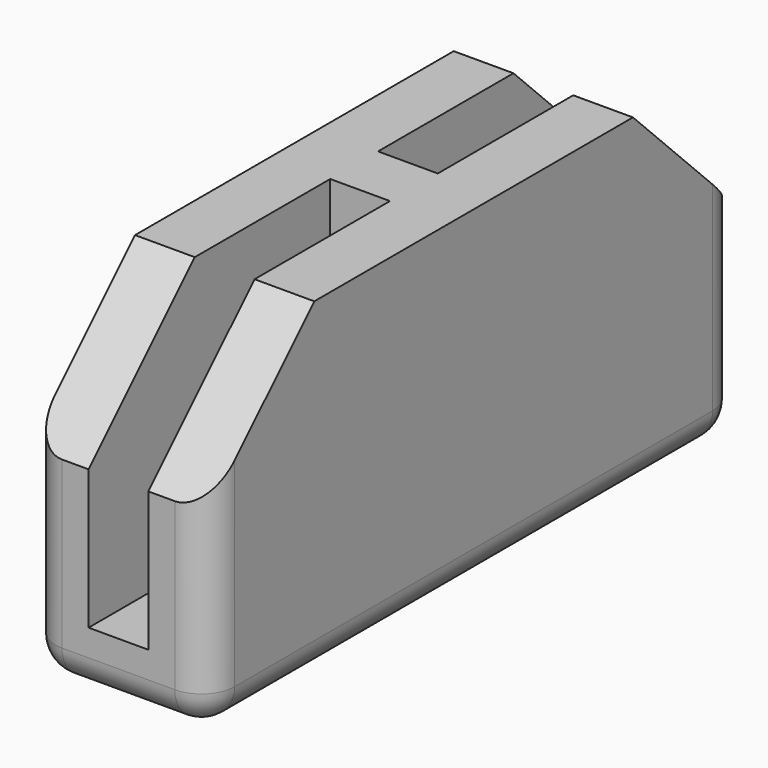
from build123d import *

# Parameters (mm, degrees)
F0_W      = 41
F0_H      = 9
F1_DEPTH  = 41
F3_DEPTH  = 9
F5_DEPTH  = 9
F7_DEPTH  = 30
F9_DEPTH  = 30
F11_DEPTH = 9
F13_DEPTH = 25
F14_R     = 1
F16_W     = 18
F16_H     = 9
F17_DEPTH = 41
F19_DEPTH = 50.001
F20_R     = 5
F21_W     = 9
F21_H     = 41
F22_DEPTH = 30
F23_W     = 27
F23_H     = 9
F24_DEPTH = 41


with BuildPart() as f1:
    # F0 (on Top) → F1 (new body)
    with BuildSketch(Plane.XY):
        Polygon((0, 50), (0, 0), (27, 0), (27, 4.5), (27, 13.5), (27, 22.5), (27, 50), (18, 50), (18, 4.5), (9, 4.5), (9, 50), align=None)
        with Locations((47.5, 9)):
            Rectangle(F0_W, F0_H)
    extrude(amount=F1_DEPTH)

    # F2 (on Top) → F3 (join)
    with BuildSketch(Plane.XY):
        Polygon((0, 50), (0, 0), (68, 0), (68, 13.5), (27, 50), align=None)
    extrude(amount=-F3_DEPTH)

    # F4 (on face) → F5 (cut, through all)
    with BuildSketch(Plane.XY):
        Polygon((56.1775657399, 18), (31.5, 39.9690524269), (31.5, 18), align=None)
    extrude(amount=-F5_DEPTH, mode=Mode.SUBTRACT)

    # F6 (on face) → F7 (cut)
    with BuildSketch(Plane(origin=(0, 0, 0), x_dir=(0, -1, 0), z_dir=(-1, 0, 0))):
        Polygon((-50, 21), (-30, 41), (-50, 41), align=None)
    extrude(amount=-F7_DEPTH, mode=Mode.SUBTRACT)

    # F8 (on face) → F9 (cut)
    with BuildSketch(Plane.XZ):
        Polygon((0, 21), (0, 41), (-20, 41), align=None)
    extrude(amount=-F9_DEPTH, mode=Mode.SUBTRACT)

    # F10 (on face) → F11 (cut, through all)
    with BuildSketch(Plane.XY):
        with BuildLine():
            Line((9, 36.5), (9, 13.5))
            ThreePointArc((9, 13.5), (10.3180194847, 10.3180194847), (13.5, 9))
            ThreePointArc((13.5, 9), (16.6819805153, 10.3180194847), (18, 13.5))
            Line((18, 13.5), (18, 36.5))
            ThreePointArc((18, 36.5), (16.6819805153, 39.6819805153), (13.5, 41))
            ThreePointArc((13.5, 41), (10.3180194847, 39.6819805153), (9, 36.5))
        make_face()
        with BuildLine():
            ThreePointArc((59, 0), (57.6819805153, 3.1819805153), (54.5, 4.5))
            Line((54.5, 4.5), (40.5, 4.5))
            ThreePointArc((40.5, 4.5), (37.3180194847, 3.1819805153), (36, 0))
            Line((36, 0), (59, 0))
        make_face()
    extrude(amount=-F11_DEPTH, mode=Mode.SUBTRACT)

    # F12 (on face) → F13 (cut)
    with BuildSketch(Plane.XZ.offset(-4.5)):
        Polygon((68, 21), (68, 41), (48, 41), align=None)
        Polygon((59, 17.2720779386), (44.2720779386, 32), (36, 32), (36, 9), (59, 9), align=None)
    extrude(amount=-F13_DEPTH, mode=Mode.SUBTRACT)

    # F14
    f14_edges = [f1.edges().sort_by_distance(p)[0] for p in [
        (31.5, 18, -4.5),
        (31.5, 39.969052, -4.5),
        (56.177566, 18, -4.5),
        (36, 9, 9),
        (36, 9, 32),
        (44.272078, 9, 32),
        (59, 9, 17.272078),
        (59, 9, 9),
    ]]
    fillet(f14_edges, radius=F14_R)

    # F15: F1 across face


with BuildPart() as f1_1:
    add(f1.part)
    add(f1.part.mirror(Plane(origin=(14.5188679245, 0, 14.8396226415), x_dir=(1, 0, 0), z_dir=(0, -1, 0))))

    # F16 (on face) → F17 (cut)
    with BuildSketch(Plane.XY.offset(41)):
        with Locations((18, 0)):
            Rectangle(F16_W, F16_H)
    extrude(amount=-F17_DEPTH, mode=Mode.SUBTRACT)

    # F18 (on face) → F19 (cut, through all)
    with BuildSketch(Plane.XY.offset(41)):
        Polygon((27, 70.5021247268), (27, -13.5), (27, -65.4299333692), (95.0682684779, -18.0513188243), (92.9595008492, 35.7407592237), align=None)
    extrude(amount=-F19_DEPTH, mode=Mode.SUBTRACT)

    # F20
    f20_edges = [f1_1.edges().sort_by_distance(p)[0] for p in [
        (27, -50, 6),
        (0, -50, 6),
        (27, 50, 6),
        (0, 50, 6),
        (0, 0, -9),
        (27, 0, -9),
        (13.5, 50, -9),
        (13.5, -50, -9),
    ]]
    fillet(f20_edges, radius=F20_R)

    # F21 (on face) → F22 (cut)
    with BuildSketch(Plane.YZ.offset(27)):
        with Locations((0, 20.5)):
            Rectangle(F21_W, F21_H)
    extrude(amount=-F22_DEPTH, mode=Mode.SUBTRACT)

    # F23 (on face) → F24 (join)
    with BuildSketch(Plane.XY):
        with Locations((13.5, 0)):
            Rectangle(F23_W, F23_H)
    extrude(amount=F24_DEPTH)


solid = f1_1.part
